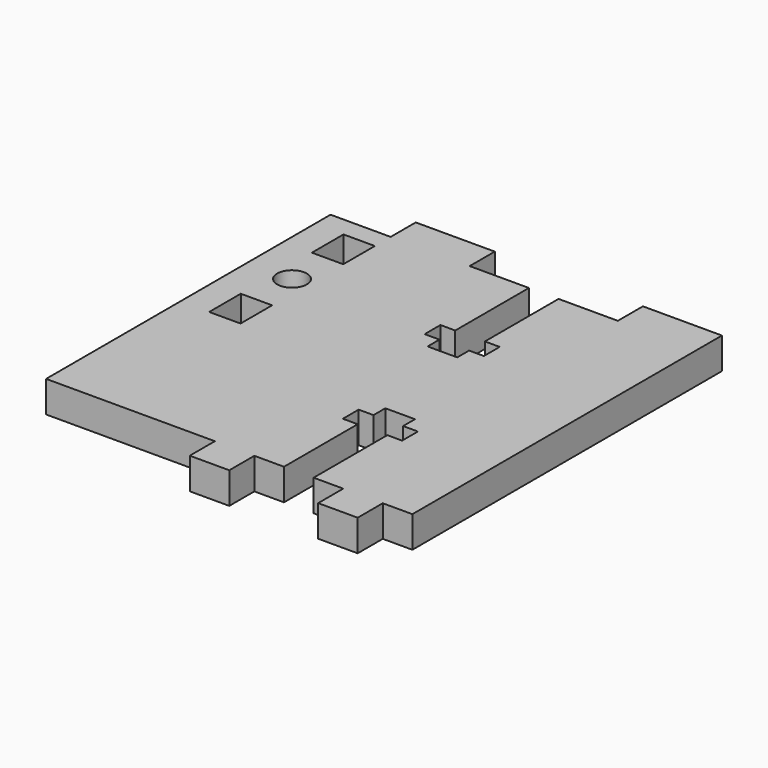
from build123d import *

# Parameters (mm, degrees)
F0_W     = 3.175
F0_H     = 4
F0_R     = 1.5
F1_DEPTH = 3.175


# Not quite as in the source:
# - a length typed as a fraction of an inch, garbled in the dataset ("3 / 203.2 mm" for 3/8 in), is restored
# - a feature names something its author has since deleted; it is built from what else it names


with BuildPart() as f1:
    # F0 (on Top) → F1 (new body)
    with BuildSketch(Plane.XY):
        Polygon((11.1548891366, 23.9696219414), (8.1548891366, 23.9696219414), (8.1548891366, 25.4696219414), (6.6548891366, 25.4696219414), (6.6548891366, 27.4696219414), (8.1548891366, 27.4696219414), (8.1548891366, 36.7946219414), (2.1548891366, 36.7946219414), (2.1548891366, 39.9696219414), (-5.8451108634, 39.9696219414), (-5.8451108634, 36.7946219414), (-11.9326108634, 36.7946219414), (-11.9326108634, 0.7946219414), (5.1548891366, 0.7946219414), (5.1548891366, -2.3803780586), (9.1548891366, -2.3803780586), (9.1548891366, 0.7946219414), (12.1548891366, 0.7946219414), (12.1548891366, 10.1196219414), (10.6548891366, 10.1196219414), (10.6548891366, 12.1196219414), (12.1548891366, 12.1196219414), (12.1548891366, 13.6196219414), (15.1548891366, 13.6196219414), (15.1548891366, 12.1196219414), (16.6548891366, 12.1196219414), (16.6548891366, 10.1196219414), (15.1548891366, 10.1196219414), (15.1548891366, 0.7946219414), (18.1548891366, 0.7946219414), (18.1548891366, -2.3803780586), (22.1548891366, -2.3803780586), (22.1548891366, 0.7946219414), (25.1548891366, 0.7946219414), (25.1548891366, 36.7946219414), (25.1548891366, 39.9696219414), (17.1548891366, 39.9696219414), (17.1548891366, 36.7946219414), (11.1548891366, 36.7946219414), (11.1548891366, 27.4696219414), (12.6548891366, 27.4696219414), (12.6548891366, 25.4696219414), (11.1548891366, 25.4696219414), align=None)
        with Locations((-7.4326108634, 19.7946219414)):
            Rectangle(F0_W, F0_H, mode=Mode.SUBTRACT)
        with Locations((-7.4326108634, 26.2946219414)):
            Circle(F0_R, mode=Mode.SUBTRACT)
        with Locations((-7.4326108634, 32.7946219414)):
            Rectangle(F0_W, F0_H, mode=Mode.SUBTRACT)
    extrude(amount=F1_DEPTH)


solid = f1.part
